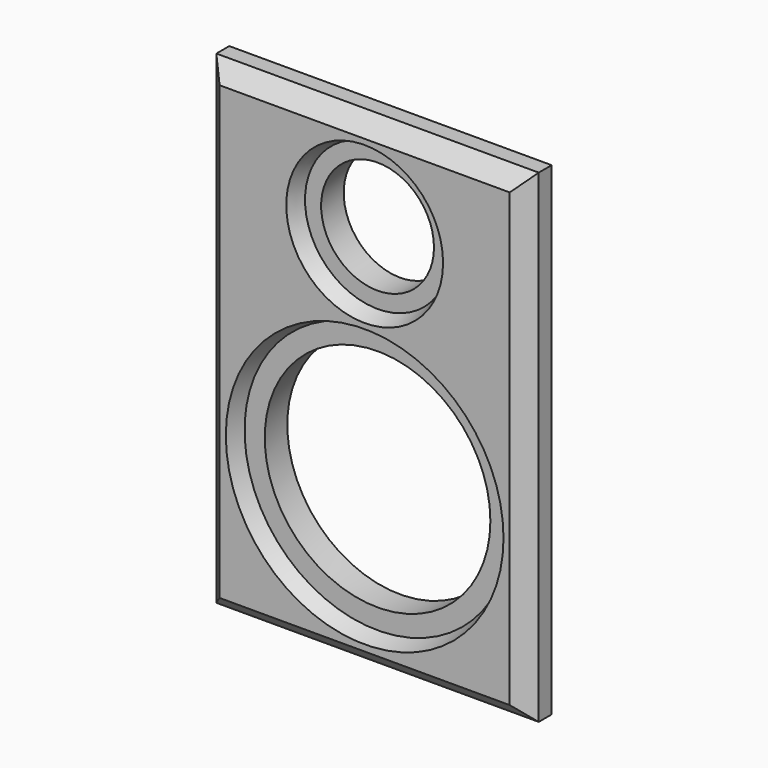
from build123d import *

# Parameters (mm, degrees)
F9_W      = 185
F9_H      = 284.8
F10_DEPTH = 7.5
F11_W     = 200
F11_H     = 300
F12_DEPTH = 20
F16_R     = 70
F17_DEPTH = 157.5
F18_R     = 82.5
F19_DEPTH = 140
F20_R     = 35
F21_DEPTH = 157.5
F22_R     = 45
F23_DEPTH = 140
F13_W     = 40
F13_H     = 300
F24_DEPTH = 200
F25_SIZE  = 10
F26_SIZE2 = 9.99999
F26_SIZE  = 3.639692
F27_SIZE2 = 9.99999
F27_SIZE  = 3.639692


# Not quite as in the source:
# - a fillet or chamfer is up to 0.001 mm smaller than in the source, because OpenCascade refuses the exact size


with BuildPart() as f10:
    # F9 (on offset) → F10 (new body)
    with BuildSketch(Plane.XZ.offset(142.5)):
        with Locations((0, 150.1)):
            Rectangle(F9_W, F9_H)
    extrude(amount=F10_DEPTH)

    # F11 (on offset) → F12 (join)
    with BuildSketch(Plane.XZ.offset(150)):
        with Locations((0, 150)):
            Rectangle(F11_W, F11_H)
    extrude(amount=F12_DEPTH)

    # F16 (on offset) → F17 (cut, through all)
    with BuildSketch(Plane.XZ.offset(300)):
        with Locations((0, 100)):
            Circle(F16_R)
    extrude(amount=-F17_DEPTH, mode=Mode.SUBTRACT)

    # F18 (on offset) → F19 (cut, through all)
    with BuildSketch(Plane.XZ.offset(300)):
        with Locations((0, 100)):
            Circle(F18_R)
    extrude(amount=-F19_DEPTH, mode=Mode.SUBTRACT)

    # F20 (on offset) → F21 (cut, through all)
    with BuildSketch(Plane.XZ.offset(300)):
        with Locations((0, 238)):
            Circle(F20_R)
    extrude(amount=-F21_DEPTH, mode=Mode.SUBTRACT)

    # F22 (on offset) → F23 (cut, through all)
    with BuildSketch(Plane.XZ.offset(300)):
        with Locations((0, 238)):
            Circle(F22_R)
    extrude(amount=-F23_DEPTH, mode=Mode.SUBTRACT)

    # F13 (on offset) → F24 (cut, through all)
    with BuildSketch(Plane.YZ.offset(100)):
        with Locations((-200, 150)):
            Rectangle(F13_W, F13_H)
    extrude(amount=-F24_DEPTH, mode=Mode.SUBTRACT)

    # F25
    f25_edges = [f10.edges().sort_by_distance(p)[0] for p in [
        (100, -170, 150),
        (0, -170, 300),
        (-100, -170, 150),
        (0, -170, 0),
    ]]
    chamfer(f25_edges, length=F25_SIZE)

    # F26 (size 3.6397023427 and 10 in the source; OpenCascade refuses exactly that, so slightly less here)
    f26_edges = [f10.edges().sort_by_distance(p)[0] for p in [
        (-82.5, -170, 100),
    ]]
    f26_side = f10.faces().sort_by_distance((86.671337, -170, 150))[0]
    chamfer(f26_edges, length=F26_SIZE, length2=F26_SIZE2, reference=f26_side)

    # F27 (size 3.6397023427 and 10 in the source; OpenCascade refuses exactly that, so slightly less here)
    f27_edges = [f10.edges().sort_by_distance(p)[0] for p in [
        (-45, -170, 238),
    ]]
    f27_side = f10.faces().sort_by_distance((-89.468355, -170, 100))[0]
    chamfer(f27_edges, length=F27_SIZE, length2=F27_SIZE2, reference=f27_side)


solid = f10.part
